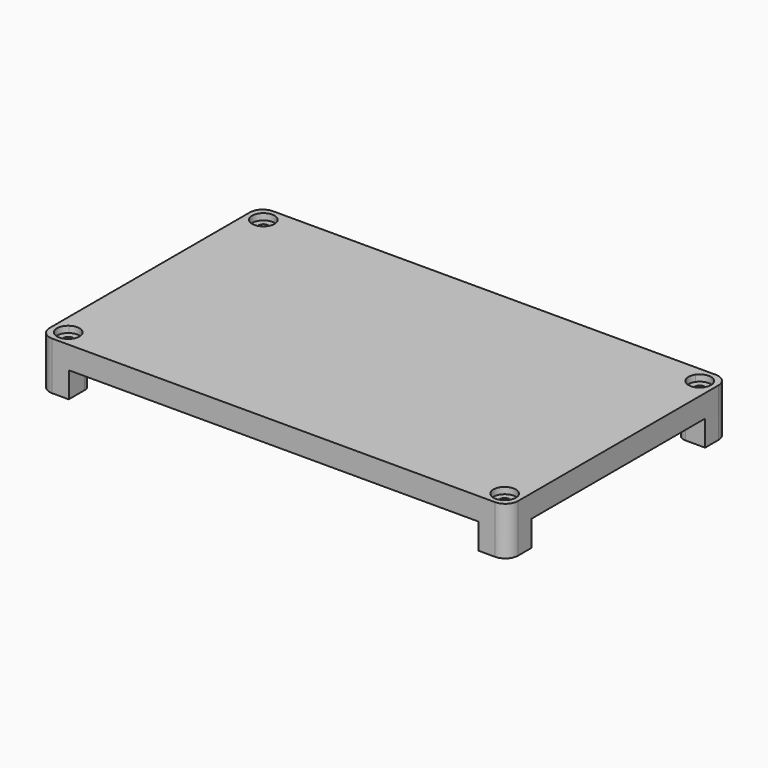
from build123d import *

# Parameters (mm, degrees)
F0_W     = 127.7
F0_H     = 3
F0_W_2   = 3
F0_H_2   = 5
F0_R     = 1.5
F0_H_3   = 6
F0_H_4   = 4
F0_H_5   = 5.7
F1_DEPTH = 2.5
F2_DEPTH = 5
F3_DEPTH = 13
F4_DEPTH = 2


with BuildPart() as f1:
    # F0 (on Top) → F1 (new body)
    with BuildSketch(Plane.XY):
        with BuildLine():
            ThreePointArc((0, 4), (1.1715728753, 1.1715728753), (4, 0))
            Line((4, 0), (9.15, 0))
            Line((9.15, 0), (9.15, 3))
            Line((9.15, 3), (7.8722813233, 3))
            ThreePointArc((7.8722813233, 3), (2.5251262658, 2.5251262658), (3, 7.8722813233))
            Line((3, 7.8722813233), (3, 9.15))
            Line((3, 9.15), (0, 9.15))
            Line((0, 9.15), (0, 4))
        make_face()
        with Locations((73, 1.5)):
            Rectangle(F0_W, F0_H)
        with BuildLine():
            Line((136.85, 3), (136.85, 0))
            Line((136.85, 0), (142, 0))
            ThreePointArc((142, 0), (144.8284271247, 1.1715728753), (146, 4))
            Line((146, 4), (146, 9.15))
            Line((146, 9.15), (143, 9.15))
            Line((143, 9.15), (143, 7.8722813233))
            ThreePointArc((143, 7.8722813233), (144.1024184115, 6.6201851746), (144.5, 5))
            ThreePointArc((144.5, 5), (142.0480971731, 1.6606149794), (138.1277186767, 3))
            Line((138.1277186767, 3), (136.85, 3))
        make_face()
        with BuildLine():
            Line((7.8722813233, 3), (9.15, 3))
            Line((9.15, 3), (9.15, 6.15))
            ThreePointArc((9.15, 6.15), (8.2713203436, 8.2713203436), (6.15, 9.15))
            Line((6.15, 9.15), (3, 9.15))
            Line((3, 9.15), (3, 7.8722813233))
            ThreePointArc((3, 7.8722813233), (6.6201851746, 8.1024184115), (8.5, 5))
            ThreePointArc((8.5, 5), (8.3393850206, 3.9519028269), (7.8722813233, 3))
        make_face()
        with Locations((1.5, 11.65)):
            Rectangle(F0_W_2, F0_H_2)
        with BuildLine():
            Line((136.85, 6.15), (136.85, 3))
            Line((136.85, 3), (138.1277186767, 3))
            ThreePointArc((138.1277186767, 3), (138.5251262658, 7.4748737342), (143, 7.8722813233))
            Line((143, 7.8722813233), (143, 9.15))
            Line((143, 9.15), (139.85, 9.15))
            ThreePointArc((139.85, 9.15), (137.7286796564, 8.2713203436), (136.85, 6.15))
        make_face()
        with BuildLine():
            ThreePointArc((3, 7.8722813233), (2.5251262658, 2.5251262658), (7.8722813233, 3))
            Line((7.8722813233, 3), (3, 3))
            Line((3, 3), (3, 7.8722813233))
        make_face()
        with BuildLine():
            Line((3, 3), (7.8722813233, 3))
            ThreePointArc((7.8722813233, 3), (8.3393850206, 3.9519028269), (8.5, 5))
            ThreePointArc((8.5, 5), (6.6201851746, 8.1024184115), (3, 7.8722813233))
            Line((3, 7.8722813233), (3, 3))
        make_face()
        with Locations((5, 5)):
            Circle(F0_R, mode=Mode.SUBTRACT)
        with Locations((1.5, 17.15)):
            Rectangle(F0_W_2, F0_H_3)
        with BuildLine():
            ThreePointArc((143, 7.8722813233), (138.5251262658, 7.4748737342), (138.1277186767, 3))
            Line((138.1277186767, 3), (143, 3))
            Line((143, 3), (143, 7.8722813233))
        make_face()
        with Locations((141, 5)):
            Circle(F0_R, mode=Mode.SUBTRACT)
        with BuildLine():
            Line((143, 3), (138.1277186767, 3))
            ThreePointArc((138.1277186767, 3), (142.0480971731, 1.6606149794), (144.5, 5))
            ThreePointArc((144.5, 5), (144.1024184115, 6.6201851746), (143, 7.8722813233))
            Line((143, 7.8722813233), (143, 3))
        make_face()
        with Locations((1.5, 22.15)):
            Rectangle(F0_W_2, F0_H_4)
        Polygon((143, 9.15), (146, 9.15), (146, 14.15), (146, 20.15), (146, 24.15), (146, 30.15), (146, 35.85), (146, 41.85), (146, 45.85), (146, 51.85), (146, 55.85), (146, 61.85), (146, 65.85), (146, 71.85), (146, 76.85), (143, 76.85), (143, 71.85), (143, 65.85), (143, 61.85), (143, 55.85), (143, 51.85), (143, 45.85), (143, 41.85), (143, 35.85), (143, 30.15), (143, 24.15), (143, 20.15), (143, 14.15), align=None)
        with Locations((1.5, 27.15)):
            Rectangle(F0_W_2, F0_H_3)
        with Locations((1.5, 33)):
            Rectangle(F0_W_2, F0_H_5)
        with Locations((1.5, 38.85)):
            Rectangle(F0_W_2, F0_H_3)
        with Locations((1.5, 43.85)):
            Rectangle(F0_W_2, F0_H_4)
        with Locations((1.5, 48.85)):
            Rectangle(F0_W_2, F0_H_3)
        with Locations((1.5, 53.85)):
            Rectangle(F0_W_2, F0_H_4)
        with Locations((1.5, 58.85)):
            Rectangle(F0_W_2, F0_H_3)
        with Locations((1.5, 63.85)):
            Rectangle(F0_W_2, F0_H_4)
        with Locations((1.5, 68.85)):
            Rectangle(F0_W_2, F0_H_3)
        with Locations((1.5, 74.35)):
            Rectangle(F0_W_2, F0_H_2)
        with BuildLine():
            Line((0, 82), (0, 76.85))
            Line((0, 76.85), (3, 76.85))
            Line((3, 76.85), (3, 78.1277186767))
            ThreePointArc((3, 78.1277186767), (2.5251262658, 83.4748737342), (7.8722813233, 83))
            Line((7.8722813233, 83), (9.15, 83))
            Line((9.15, 83), (9.15, 86))
            Line((9.15, 86), (4, 86))
            ThreePointArc((4, 86), (1.1715728753, 84.8284271247), (0, 82))
        make_face()
        with BuildLine():
            Line((3, 78.1277186767), (3, 76.85))
            Line((3, 76.85), (6.15, 76.85))
            ThreePointArc((6.15, 76.85), (8.2713203436, 77.7286796564), (9.15, 79.85))
            Line((9.15, 79.85), (9.15, 83))
            Line((9.15, 83), (7.8722813233, 83))
            ThreePointArc((7.8722813233, 83), (8.3393850206, 82.0480971731), (8.5, 81))
            ThreePointArc((8.5, 81), (6.6201851746, 77.8975815885), (3, 78.1277186767))
        make_face()
        with BuildLine():
            ThreePointArc((7.8722813233, 83), (2.5251262658, 83.4748737342), (3, 78.1277186767))
            Line((3, 78.1277186767), (3, 83))
            Line((3, 83), (7.8722813233, 83))
        make_face()
        with BuildLine():
            Line((3, 83), (3, 78.1277186767))
            ThreePointArc((3, 78.1277186767), (6.6201851746, 77.8975815885), (8.5, 81))
            ThreePointArc((8.5, 81), (8.3393850206, 82.0480971731), (7.8722813233, 83))
            Line((7.8722813233, 83), (3, 83))
        make_face()
        with Locations((5, 81)):
            Circle(F0_R, mode=Mode.SUBTRACT)
        with BuildLine():
            Line((143, 76.85), (146, 76.85))
            Line((146, 76.85), (146, 82))
            ThreePointArc((146, 82), (144.8284271247, 84.8284271247), (142, 86))
            Line((142, 86), (136.85, 86))
            Line((136.85, 86), (136.85, 83))
            Line((136.85, 83), (138.1277186767, 83))
            ThreePointArc((138.1277186767, 83), (142.0480971731, 84.3393850206), (144.5, 81))
            ThreePointArc((144.5, 81), (144.1024184115, 79.3798148254), (143, 78.1277186767))
            Line((143, 78.1277186767), (143, 76.85))
        make_face()
        with Locations((73, 84.5)):
            Rectangle(F0_W, F0_H)
        with BuildLine():
            Line((139.85, 76.85), (143, 76.85))
            Line((143, 76.85), (143, 78.1277186767))
            ThreePointArc((143, 78.1277186767), (138.5251262658, 78.5251262658), (138.1277186767, 83))
            Line((138.1277186767, 83), (136.85, 83))
            Line((136.85, 83), (136.85, 79.85))
            ThreePointArc((136.85, 79.85), (137.7286796564, 77.7286796564), (139.85, 76.85))
        make_face()
        with BuildLine():
            ThreePointArc((138.1277186767, 83), (138.5251262658, 78.5251262658), (143, 78.1277186767))
            Line((143, 78.1277186767), (143, 83))
            Line((143, 83), (138.1277186767, 83))
        make_face()
        with Locations((141, 81)):
            Circle(F0_R, mode=Mode.SUBTRACT)
        with BuildLine():
            Line((143, 83), (143, 78.1277186767))
            ThreePointArc((143, 78.1277186767), (144.1024184115, 79.3798148254), (144.5, 81))
            ThreePointArc((144.5, 81), (142.0480971731, 84.3393850206), (138.1277186767, 83))
            Line((138.1277186767, 83), (143, 83))
        make_face()
    extrude(amount=-F1_DEPTH)

    # F0 (on Top) → F2 (join)
    with BuildSketch(Plane.XY):
        with BuildLine():
            ThreePointArc((0, 4), (1.1715728753, 1.1715728753), (4, 0))
            Line((4, 0), (9.15, 0))
            Line((9.15, 0), (9.15, 3))
            Line((9.15, 3), (7.8722813233, 3))
            ThreePointArc((7.8722813233, 3), (2.5251262658, 2.5251262658), (3, 7.8722813233))
            Line((3, 7.8722813233), (3, 9.15))
            Line((3, 9.15), (0, 9.15))
            Line((0, 9.15), (0, 4))
        make_face()
        with Locations((73, 1.5)):
            Rectangle(F0_W, F0_H)
        with BuildLine():
            Line((136.85, 3), (136.85, 0))
            Line((136.85, 0), (142, 0))
            ThreePointArc((142, 0), (144.8284271247, 1.1715728753), (146, 4))
            Line((146, 4), (146, 9.15))
            Line((146, 9.15), (143, 9.15))
            Line((143, 9.15), (143, 7.8722813233))
            ThreePointArc((143, 7.8722813233), (144.1024184115, 6.6201851746), (144.5, 5))
            ThreePointArc((144.5, 5), (142.0480971731, 1.6606149794), (138.1277186767, 3))
            Line((138.1277186767, 3), (136.85, 3))
        make_face()
        with Locations((1.5, 11.65)):
            Rectangle(F0_W_2, F0_H_2)
        with BuildLine():
            ThreePointArc((3, 7.8722813233), (2.5251262658, 2.5251262658), (7.8722813233, 3))
            Line((7.8722813233, 3), (3, 3))
            Line((3, 3), (3, 7.8722813233))
        make_face()
        with BuildLine():
            Line((3, 3), (7.8722813233, 3))
            ThreePointArc((7.8722813233, 3), (8.3393850206, 3.9519028269), (8.5, 5))
            ThreePointArc((8.5, 5), (6.6201851746, 8.1024184115), (3, 7.8722813233))
            Line((3, 7.8722813233), (3, 3))
        make_face()
        with Locations((5, 5)):
            Circle(F0_R, mode=Mode.SUBTRACT)
        with BuildLine():
            ThreePointArc((143, 7.8722813233), (138.5251262658, 7.4748737342), (138.1277186767, 3))
            Line((138.1277186767, 3), (143, 3))
            Line((143, 3), (143, 7.8722813233))
        make_face()
        with Locations((141, 5)):
            Circle(F0_R, mode=Mode.SUBTRACT)
        with BuildLine():
            Line((143, 3), (138.1277186767, 3))
            ThreePointArc((138.1277186767, 3), (142.0480971731, 1.6606149794), (144.5, 5))
            ThreePointArc((144.5, 5), (144.1024184115, 6.6201851746), (143, 7.8722813233))
            Line((143, 7.8722813233), (143, 3))
        make_face()
        with Locations((1.5, 22.15)):
            Rectangle(F0_W_2, F0_H_4)
        Polygon((143, 9.15), (146, 9.15), (146, 14.15), (146, 20.15), (146, 24.15), (146, 30.15), (146, 35.85), (146, 41.85), (146, 45.85), (146, 51.85), (146, 55.85), (146, 61.85), (146, 65.85), (146, 71.85), (146, 76.85), (143, 76.85), (143, 71.85), (143, 65.85), (143, 61.85), (143, 55.85), (143, 51.85), (143, 45.85), (143, 41.85), (143, 35.85), (143, 30.15), (143, 24.15), (143, 20.15), (143, 14.15), align=None)
        with Locations((1.5, 33)):
            Rectangle(F0_W_2, F0_H_5)
        with Locations((1.5, 43.85)):
            Rectangle(F0_W_2, F0_H_4)
        with Locations((1.5, 53.85)):
            Rectangle(F0_W_2, F0_H_4)
        with Locations((1.5, 63.85)):
            Rectangle(F0_W_2, F0_H_4)
        with Locations((1.5, 74.35)):
            Rectangle(F0_W_2, F0_H_2)
        with BuildLine():
            Line((0, 82), (0, 76.85))
            Line((0, 76.85), (3, 76.85))
            Line((3, 76.85), (3, 78.1277186767))
            ThreePointArc((3, 78.1277186767), (2.5251262658, 83.4748737342), (7.8722813233, 83))
            Line((7.8722813233, 83), (9.15, 83))
            Line((9.15, 83), (9.15, 86))
            Line((9.15, 86), (4, 86))
            ThreePointArc((4, 86), (1.1715728753, 84.8284271247), (0, 82))
        make_face()
        with BuildLine():
            ThreePointArc((7.8722813233, 83), (2.5251262658, 83.4748737342), (3, 78.1277186767))
            Line((3, 78.1277186767), (3, 83))
            Line((3, 83), (7.8722813233, 83))
        make_face()
        with BuildLine():
            Line((3, 83), (3, 78.1277186767))
            ThreePointArc((3, 78.1277186767), (6.6201851746, 77.8975815885), (8.5, 81))
            ThreePointArc((8.5, 81), (8.3393850206, 82.0480971731), (7.8722813233, 83))
            Line((7.8722813233, 83), (3, 83))
        make_face()
        with Locations((5, 81)):
            Circle(F0_R, mode=Mode.SUBTRACT)
        with BuildLine():
            Line((143, 76.85), (146, 76.85))
            Line((146, 76.85), (146, 82))
            ThreePointArc((146, 82), (144.8284271247, 84.8284271247), (142, 86))
            Line((142, 86), (136.85, 86))
            Line((136.85, 86), (136.85, 83))
            Line((136.85, 83), (138.1277186767, 83))
            ThreePointArc((138.1277186767, 83), (142.0480971731, 84.3393850206), (144.5, 81))
            ThreePointArc((144.5, 81), (144.1024184115, 79.3798148254), (143, 78.1277186767))
            Line((143, 78.1277186767), (143, 76.85))
        make_face()
        with Locations((73, 84.5)):
            Rectangle(F0_W, F0_H)
        with BuildLine():
            ThreePointArc((138.1277186767, 83), (138.5251262658, 78.5251262658), (143, 78.1277186767))
            Line((143, 78.1277186767), (143, 83))
            Line((143, 83), (138.1277186767, 83))
        make_face()
        with Locations((141, 81)):
            Circle(F0_R, mode=Mode.SUBTRACT)
        with BuildLine():
            Line((143, 83), (143, 78.1277186767))
            ThreePointArc((143, 78.1277186767), (144.1024184115, 79.3798148254), (144.5, 81))
            ThreePointArc((144.5, 81), (142.0480971731, 84.3393850206), (138.1277186767, 83))
            Line((138.1277186767, 83), (143, 83))
        make_face()
    extrude(amount=-F2_DEPTH)

    # F0 (on Top) → F3 (join)
    with BuildSketch(Plane.XY):
        with BuildLine():
            Line((7.8722813233, 3), (9.15, 3))
            Line((9.15, 3), (9.15, 6.15))
            ThreePointArc((9.15, 6.15), (8.2713203436, 8.2713203436), (6.15, 9.15))
            Line((6.15, 9.15), (3, 9.15))
            Line((3, 9.15), (3, 7.8722813233))
            ThreePointArc((3, 7.8722813233), (6.6201851746, 8.1024184115), (8.5, 5))
            ThreePointArc((8.5, 5), (8.3393850206, 3.9519028269), (7.8722813233, 3))
        make_face()
        with BuildLine():
            Line((3, 78.1277186767), (3, 76.85))
            Line((3, 76.85), (6.15, 76.85))
            ThreePointArc((6.15, 76.85), (8.2713203436, 77.7286796564), (9.15, 79.85))
            Line((9.15, 79.85), (9.15, 83))
            Line((9.15, 83), (7.8722813233, 83))
            ThreePointArc((7.8722813233, 83), (8.3393850206, 82.0480971731), (8.5, 81))
            ThreePointArc((8.5, 81), (6.6201851746, 77.8975815885), (3, 78.1277186767))
        make_face()
        with BuildLine():
            Line((139.85, 76.85), (143, 76.85))
            Line((143, 76.85), (143, 78.1277186767))
            ThreePointArc((143, 78.1277186767), (138.5251262658, 78.5251262658), (138.1277186767, 83))
            Line((138.1277186767, 83), (136.85, 83))
            Line((136.85, 83), (136.85, 79.85))
            ThreePointArc((136.85, 79.85), (137.7286796564, 77.7286796564), (139.85, 76.85))
        make_face()
        with BuildLine():
            Line((136.85, 6.15), (136.85, 3))
            Line((136.85, 3), (138.1277186767, 3))
            ThreePointArc((138.1277186767, 3), (138.5251262658, 7.4748737342), (143, 7.8722813233))
            Line((143, 7.8722813233), (143, 9.15))
            Line((143, 9.15), (139.85, 9.15))
            ThreePointArc((139.85, 9.15), (137.7286796564, 8.2713203436), (136.85, 6.15))
        make_face()
        with BuildLine():
            Line((136.85, 3), (136.85, 0))
            Line((136.85, 0), (142, 0))
            ThreePointArc((142, 0), (144.8284271247, 1.1715728753), (146, 4))
            Line((146, 4), (146, 9.15))
            Line((146, 9.15), (143, 9.15))
            Line((143, 9.15), (143, 7.8722813233))
            ThreePointArc((143, 7.8722813233), (144.1024184115, 6.6201851746), (144.5, 5))
            ThreePointArc((144.5, 5), (142.0480971731, 1.6606149794), (138.1277186767, 3))
            Line((138.1277186767, 3), (136.85, 3))
        make_face()
        with BuildLine():
            Line((143, 76.85), (146, 76.85))
            Line((146, 76.85), (146, 82))
            ThreePointArc((146, 82), (144.8284271247, 84.8284271247), (142, 86))
            Line((142, 86), (136.85, 86))
            Line((136.85, 86), (136.85, 83))
            Line((136.85, 83), (138.1277186767, 83))
            ThreePointArc((138.1277186767, 83), (142.0480971731, 84.3393850206), (144.5, 81))
            ThreePointArc((144.5, 81), (144.1024184115, 79.3798148254), (143, 78.1277186767))
            Line((143, 78.1277186767), (143, 76.85))
        make_face()
        with BuildLine():
            Line((0, 82), (0, 76.85))
            Line((0, 76.85), (3, 76.85))
            Line((3, 76.85), (3, 78.1277186767))
            ThreePointArc((3, 78.1277186767), (2.5251262658, 83.4748737342), (7.8722813233, 83))
            Line((7.8722813233, 83), (9.15, 83))
            Line((9.15, 83), (9.15, 86))
            Line((9.15, 86), (4, 86))
            ThreePointArc((4, 86), (1.1715728753, 84.8284271247), (0, 82))
        make_face()
        with BuildLine():
            ThreePointArc((0, 4), (1.1715728753, 1.1715728753), (4, 0))
            Line((4, 0), (9.15, 0))
            Line((9.15, 0), (9.15, 3))
            Line((9.15, 3), (7.8722813233, 3))
            ThreePointArc((7.8722813233, 3), (2.5251262658, 2.5251262658), (3, 7.8722813233))
            Line((3, 7.8722813233), (3, 9.15))
            Line((3, 9.15), (0, 9.15))
            Line((0, 9.15), (0, 4))
        make_face()
    extrude(amount=-F3_DEPTH)

    # F0 (on Top) → F4 (join)
    with BuildSketch(Plane.XY):
        with BuildLine():
            Line((0, 82), (0, 76.85))
            Line((0, 76.85), (3, 76.85))
            Line((3, 76.85), (3, 78.1277186767))
            ThreePointArc((3, 78.1277186767), (2.5251262658, 83.4748737342), (7.8722813233, 83))
            Line((7.8722813233, 83), (9.15, 83))
            Line((9.15, 83), (9.15, 86))
            Line((9.15, 86), (4, 86))
            ThreePointArc((4, 86), (1.1715728753, 84.8284271247), (0, 82))
        make_face()
        with Locations((73, 84.5)):
            Rectangle(F0_W, F0_H)
        with BuildLine():
            Line((143, 76.85), (146, 76.85))
            Line((146, 76.85), (146, 82))
            ThreePointArc((146, 82), (144.8284271247, 84.8284271247), (142, 86))
            Line((142, 86), (136.85, 86))
            Line((136.85, 86), (136.85, 83))
            Line((136.85, 83), (138.1277186767, 83))
            ThreePointArc((138.1277186767, 83), (142.0480971731, 84.3393850206), (144.5, 81))
            ThreePointArc((144.5, 81), (144.1024184115, 79.3798148254), (143, 78.1277186767))
            Line((143, 78.1277186767), (143, 76.85))
        make_face()
        with BuildLine():
            Line((3, 78.1277186767), (3, 76.85))
            Line((3, 76.85), (6.15, 76.85))
            ThreePointArc((6.15, 76.85), (8.2713203436, 77.7286796564), (9.15, 79.85))
            Line((9.15, 79.85), (9.15, 83))
            Line((9.15, 83), (7.8722813233, 83))
            ThreePointArc((7.8722813233, 83), (8.3393850206, 82.0480971731), (8.5, 81))
            ThreePointArc((8.5, 81), (6.6201851746, 77.8975815885), (3, 78.1277186767))
        make_face()
        with BuildLine():
            ThreePointArc((0, 4), (1.1715728753, 1.1715728753), (4, 0))
            Line((4, 0), (9.15, 0))
            Line((9.15, 0), (9.15, 3))
            Line((9.15, 3), (7.8722813233, 3))
            ThreePointArc((7.8722813233, 3), (2.5251262658, 2.5251262658), (3, 7.8722813233))
            Line((3, 7.8722813233), (3, 9.15))
            Line((3, 9.15), (0, 9.15))
            Line((0, 9.15), (0, 4))
        make_face()
        with Locations((1.5, 11.65)):
            Rectangle(F0_W_2, F0_H_2)
        with Locations((1.5, 22.15)):
            Rectangle(F0_W_2, F0_H_4)
        with Locations((1.5, 33)):
            Rectangle(F0_W_2, F0_H_5)
        with Locations((1.5, 43.85)):
            Rectangle(F0_W_2, F0_H_4)
        with Locations((1.5, 53.85)):
            Rectangle(F0_W_2, F0_H_4)
        with Locations((1.5, 63.85)):
            Rectangle(F0_W_2, F0_H_4)
        with Locations((1.5, 74.35)):
            Rectangle(F0_W_2, F0_H_2)
        with BuildLine():
            Line((9.15, 6.15), (9.15, 3))
            Line((9.15, 3), (136.85, 3))
            Line((136.85, 3), (136.85, 6.15))
            ThreePointArc((136.85, 6.15), (137.7286796564, 8.2713203436), (139.85, 9.15))
            Line((139.85, 9.15), (143, 9.15))
            Line((143, 9.15), (143, 14.15))
            Line((143, 14.15), (143, 20.15))
            Line((143, 20.15), (143, 24.15))
            Line((143, 24.15), (143, 30.15))
            Line((143, 30.15), (143, 35.85))
            Line((143, 35.85), (143, 41.85))
            Line((143, 41.85), (143, 45.85))
            Line((143, 45.85), (143, 51.85))
            Line((143, 51.85), (143, 55.85))
            Line((143, 55.85), (143, 61.85))
            Line((143, 61.85), (143, 65.85))
            Line((143, 65.85), (143, 71.85))
            Line((143, 71.85), (143, 76.85))
            Line((143, 76.85), (139.85, 76.85))
            ThreePointArc((139.85, 76.85), (137.7286796564, 77.7286796564), (136.85, 79.85))
            Line((136.85, 79.85), (136.85, 83))
            Line((136.85, 83), (9.15, 83))
            Line((9.15, 83), (9.15, 79.85))
            ThreePointArc((9.15, 79.85), (8.2713203436, 77.7286796564), (6.15, 76.85))
            Line((6.15, 76.85), (3, 76.85))
            Line((3, 76.85), (3, 71.85))
            Line((3, 71.85), (3, 65.85))
            Line((3, 65.85), (3, 61.85))
            Line((3, 61.85), (3, 55.85))
            Line((3, 55.85), (3, 51.85))
            Line((3, 51.85), (3, 45.85))
            Line((3, 45.85), (3, 41.85))
            Line((3, 41.85), (3, 35.85))
            Line((3, 35.85), (3, 30.15))
            Line((3, 30.15), (3, 24.15))
            Line((3, 24.15), (3, 20.15))
            Line((3, 20.15), (3, 14.15))
            Line((3, 14.15), (3, 9.15))
            Line((3, 9.15), (6.15, 9.15))
            ThreePointArc((6.15, 9.15), (8.2713203436, 8.2713203436), (9.15, 6.15))
        make_face()
        with BuildLine():
            Line((139.85, 76.85), (143, 76.85))
            Line((143, 76.85), (143, 78.1277186767))
            ThreePointArc((143, 78.1277186767), (138.5251262658, 78.5251262658), (138.1277186767, 83))
            Line((138.1277186767, 83), (136.85, 83))
            Line((136.85, 83), (136.85, 79.85))
            ThreePointArc((136.85, 79.85), (137.7286796564, 77.7286796564), (139.85, 76.85))
        make_face()
        with BuildLine():
            Line((136.85, 6.15), (136.85, 3))
            Line((136.85, 3), (138.1277186767, 3))
            ThreePointArc((138.1277186767, 3), (138.5251262658, 7.4748737342), (143, 7.8722813233))
            Line((143, 7.8722813233), (143, 9.15))
            Line((143, 9.15), (139.85, 9.15))
            ThreePointArc((139.85, 9.15), (137.7286796564, 8.2713203436), (136.85, 6.15))
        make_face()
        with Locations((73, 1.5)):
            Rectangle(F0_W, F0_H)
        with BuildLine():
            Line((136.85, 3), (136.85, 0))
            Line((136.85, 0), (142, 0))
            ThreePointArc((142, 0), (144.8284271247, 1.1715728753), (146, 4))
            Line((146, 4), (146, 9.15))
            Line((146, 9.15), (143, 9.15))
            Line((143, 9.15), (143, 7.8722813233))
            ThreePointArc((143, 7.8722813233), (144.1024184115, 6.6201851746), (144.5, 5))
            ThreePointArc((144.5, 5), (142.0480971731, 1.6606149794), (138.1277186767, 3))
            Line((138.1277186767, 3), (136.85, 3))
        make_face()
        Polygon((143, 9.15), (146, 9.15), (146, 14.15), (146, 20.15), (146, 24.15), (146, 30.15), (146, 35.85), (146, 41.85), (146, 45.85), (146, 51.85), (146, 55.85), (146, 61.85), (146, 65.85), (146, 71.85), (146, 76.85), (143, 76.85), (143, 71.85), (143, 65.85), (143, 61.85), (143, 55.85), (143, 51.85), (143, 45.85), (143, 41.85), (143, 35.85), (143, 30.15), (143, 24.15), (143, 20.15), (143, 14.15), align=None)
        with BuildLine():
            Line((7.8722813233, 3), (9.15, 3))
            Line((9.15, 3), (9.15, 6.15))
            ThreePointArc((9.15, 6.15), (8.2713203436, 8.2713203436), (6.15, 9.15))
            Line((6.15, 9.15), (3, 9.15))
            Line((3, 9.15), (3, 7.8722813233))
            ThreePointArc((3, 7.8722813233), (6.6201851746, 8.1024184115), (8.5, 5))
            ThreePointArc((8.5, 5), (8.3393850206, 3.9519028269), (7.8722813233, 3))
        make_face()
        with Locations((1.5, 68.85)):
            Rectangle(F0_W_2, F0_H_3)
        with Locations((1.5, 58.85)):
            Rectangle(F0_W_2, F0_H_3)
        with Locations((1.5, 48.85)):
            Rectangle(F0_W_2, F0_H_3)
        with Locations((1.5, 38.85)):
            Rectangle(F0_W_2, F0_H_3)
        with Locations((1.5, 27.15)):
            Rectangle(F0_W_2, F0_H_3)
        with Locations((1.5, 17.15)):
            Rectangle(F0_W_2, F0_H_3)
    extrude(amount=F4_DEPTH)


solid = f1.part
